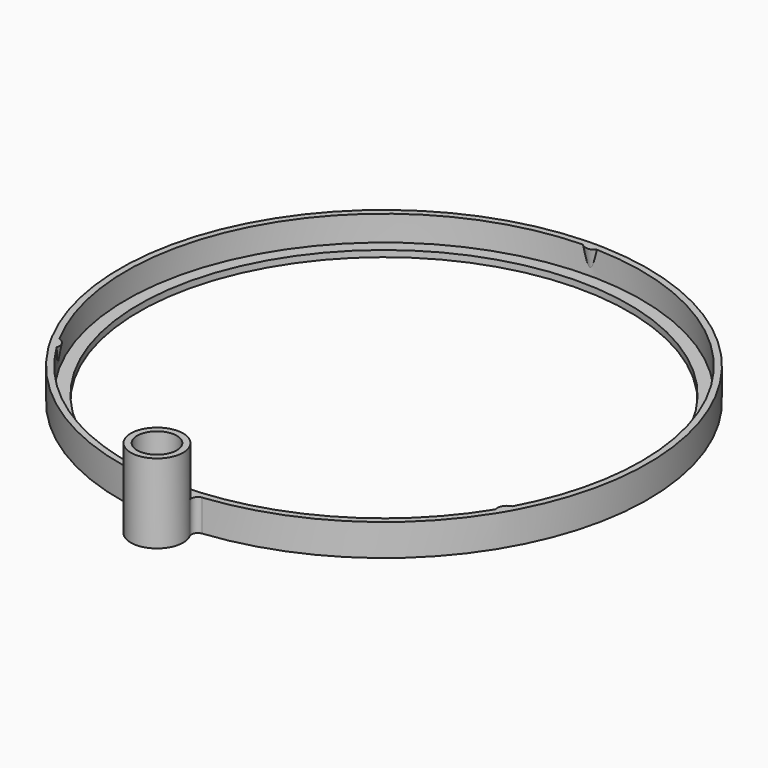
from build123d import *

# Parameters (mm, degrees)
F2_R                     = 4.191
F2_R_2                   = 3.175
F3_DEPTH                 = 12.7
F4_R                     = 1.016
F6_DEPTH                 = 3.048
DRAFT_F6_DRAFTED_ANGLE   = 10
DRAFT_F6_2_DRAFTED_ANGLE = 10
DRAFT_F6_3_DRAFTED_ANGLE = 10


# Not quite as in the source:
# - an extrude with a draft is written as a straight extrude whose walls are then drafted


with BuildPart() as f1:
    # F0 (on Front) → F1 (revolve)
    with BuildSketch(Plane.XZ):
        Polygon((39.243, 1.016), (39.243, 0), (42.291, 0), (42.291, 5.08), (41.275, 5.08), (41.275, 1.016), align=None)
    revolve(axis=Axis((0, 0, 3.1514798096), (0, 0, 1)))

    # F2 (on Top) → F3 (join)
    with BuildSketch(Plane.XY):
        with Locations((0, -45.466)):
            Circle(F2_R)
        with Locations((0, -45.466)):
            Circle(F2_R_2, mode=Mode.SUBTRACT)
    extrude(amount=F3_DEPTH)

    # F4
    f4_edges = [f1.edges().sort_by_distance(p)[0] for p in [
        (2.637132, -42.208698, 2.54),
        (-2.637132, -42.208698, 2.54),
    ]]
    fillet(f4_edges, radius=F4_R)


with BuildPart() as f6_drafted:
    # F5 (on face) → F6 (new body)
    with BuildSketch(Plane.XY.offset(5.08)):
        with BuildLine():
            ThreePointArc((1.5237525974, 42.2635405405), (0, 42.291), (-1.5237525974, 42.2635405405))
            ThreePointArc((-1.5237525974, 42.2635405405), (0, 40.767), (1.5237525974, 42.2635405405))
        make_face()
    extrude(amount=-F6_DEPTH)

    # draft_F6_drafted
    draft_f6_drafted_walls = [f6_drafted.faces().sort_by_distance(p)[0] for p in [
        (0, 42.291, 3.048),
        (0, 40.767, 3.048),
    ]]
    draft(draft_f6_drafted_walls, neutral_plane=Plane(origin=(0, 0, 5.08), x_dir=(1, 0, 0), z_dir=(0, 0, -1)), angle=DRAFT_F6_DRAFTED_ANGLE)


with BuildPart() as f1_1:
    add(f1.part)

    # join_F6_drafted: union F6_drafted
    add(f6_drafted.part)


with BuildPart() as f6_2_drafted:
    # F5 (on face) → F6, piece 2 (new body)
    with BuildSketch(Plane.XY.offset(5.08)):
        with BuildLine():
            ThreePointArc((-37.3631760607, -19.8121618118), (-36.6250803514, -21.1455), (-35.8394234633, -22.4513787287))
            ThreePointArc((-35.8394234633, -22.4513787287), (-35.3052576361, -20.3835), (-37.3631760607, -19.8121618118))
        make_face()
    extrude(amount=-F6_DEPTH)

    # draft_F6_2_drafted
    draft_f6_2_drafted_walls = [f6_2_drafted.faces().sort_by_distance(p)[0] for p in [
        (-36.6250803514, -21.1455, 3.048),
        (-35.3052576361, -20.3835, 3.048),
    ]]
    draft(draft_f6_2_drafted_walls, neutral_plane=Plane(origin=(0, 0, 5.08), x_dir=(1, 0, 0), z_dir=(0, 0, -1)), angle=DRAFT_F6_2_DRAFTED_ANGLE)


with BuildPart() as f1_2:
    add(f1_1.part)

    # join_F6_2_drafted: union F6_2_drafted
    add(f6_2_drafted.part)


with BuildPart() as f6_3_drafted:
    # F5 (on face) → F6, piece 3 (new body)
    with BuildSketch(Plane.XY.offset(5.08)):
        with BuildLine():
            ThreePointArc((35.8394234633, -22.4513787287), (36.6250803514, -21.1455), (37.3631760607, -19.8121618118))
            ThreePointArc((37.3631760607, -19.8121618118), (35.3052576361, -20.3835), (35.8394234633, -22.4513787287))
        make_face()
    extrude(amount=-F6_DEPTH)

    # draft_F6_3_drafted
    draft_f6_3_drafted_walls = [f6_3_drafted.faces().sort_by_distance(p)[0] for p in [
        (36.6250803514, -21.1455, 3.048),
        (35.3052576361, -20.3835, 3.048),
    ]]
    draft(draft_f6_3_drafted_walls, neutral_plane=Plane(origin=(0, 0, 5.08), x_dir=(1, 0, 0), z_dir=(0, 0, -1)), angle=DRAFT_F6_3_DRAFTED_ANGLE)


with BuildPart() as f1_3:
    add(f1_2.part)

    # join_F6_3_drafted: union F6_3_drafted
    add(f6_3_drafted.part)


solid = f1_3.part
